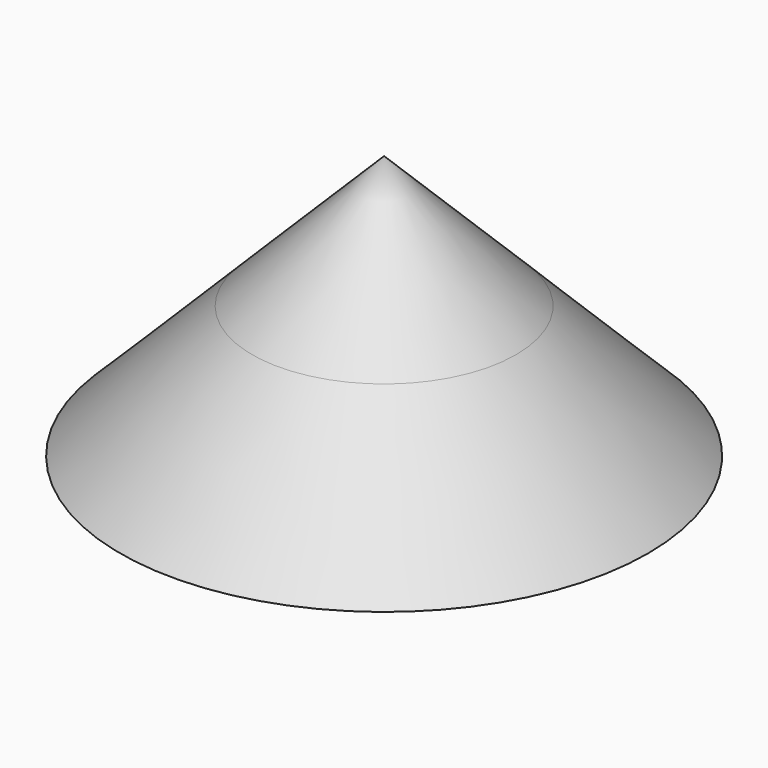
from build123d import *

# Parameters (mm, degrees)
F0_R          = 25.4
F1_DEPTH      = 25.4
F1_TAPER      = 45
F1_DEPTH_BACK = 25.4
F1_TAPER_BACK = -45


# Not quite as in the source:
# - a feature names something its author has since deleted; it is built from what else it names


with BuildPart() as f1:
    # F0 (on Top) → F1 (new body, two sides)
    with BuildSketch(Plane.XY) as f1_sk:
        Circle(F0_R)
    extrude(amount=F1_DEPTH, taper=F1_TAPER)
    extrude(f1_sk.sketch, amount=-F1_DEPTH_BACK, taper=F1_TAPER_BACK)


solid = f1.part
